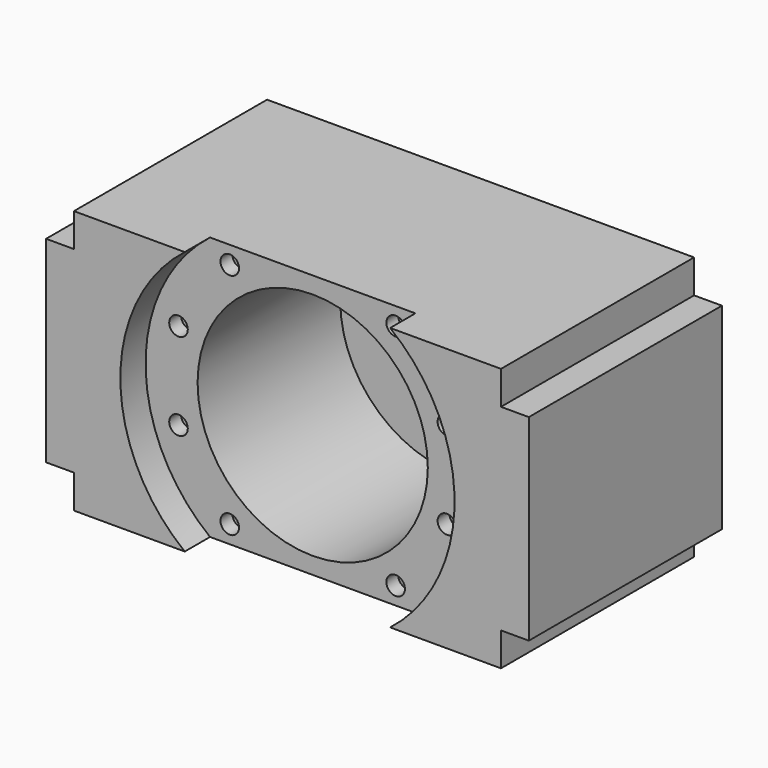
from build123d import *

# Parameters (mm, degrees)
F0_R     = 124
F1_DEPTH = 260
F2_R     = 124
F3_DEPTH = 34
F4_R     = 124
F5_DEPTH = 34
F6_R     = 10
F7_DEPTH = 16


with BuildPart() as f1:
    # F0 (on Front) → F1 (new body)
    with BuildSketch(Plane.XZ):
        Polygon((490, 0), (30, 0), (30, -36), (0, -36), (0, -248), (30, -248), (30, -284), (490, -284), (490, -248), (520, -248), (520, -36), (490, -36), align=None)
        with Locations((260, -142)):
            Circle(F0_R, mode=Mode.SUBTRACT)
    extrude(amount=F1_DEPTH)

    # F2 (on face) → F3 (cut)
    with BuildSketch(Plane.XZ.offset(260)):
        with BuildLine():
            Line((149.3835455278, -284), (370.6164544722, -284))
            ThreePointArc((370.6164544722, -284), (440, -142), (370.6164544722, 0))
            Line((370.6164544722, 0), (149.3835455278, 0))
            ThreePointArc((149.3835455278, 0), (80, -142), (149.3835455278, -284))
        make_face()
        with Locations((260, -142)):
            Circle(F2_R, mode=Mode.SUBTRACT)
    extrude(amount=-F3_DEPTH, mode=Mode.SUBTRACT)

    # F4 (on face) → F5 (join)
    with BuildSketch(Plane(origin=(0, 0, 0), x_dir=(-1, 0, 0), z_dir=(0, 1, 0))):
        Polygon((-30, -36), (-30, 0), (-490, 0), (-490, -36), (-520, -36), (-520, -248), (-490, -248), (-490, -284), (-30, -284), (-30, -248), (0, -248), (0, -36), align=None)
        with Locations((-260, -142)):
            Circle(F4_R, mode=Mode.SUBTRACT)
        with Locations((-260, -142)):
            Circle(F4_R)
    extrude(amount=-F5_DEPTH)

    # F6 (on face) → F7 (cut)
    with BuildSketch(Plane.XZ.offset(226)):
        with Locations((170.6566416515, -19.029416855)):
            Circle(F6_R)
        with Locations((115.4394095231, -95.029416855)):
            Circle(F6_R)
        with Locations((115.4394095231, -188.970583145)):
            Circle(F6_R)
        with Locations((170.6566416515, -264.970583145)):
            Circle(F6_R)
        with Locations((349.3433583485, -264.970583145)):
            Circle(F6_R)
        with Locations((404.5605904769, -188.970583145)):
            Circle(F6_R)
        with Locations((404.5605904769, -95.029416855)):
            Circle(F6_R)
        with Locations((349.3433583485, -19.029416855)):
            Circle(F6_R)
    extrude(amount=-F7_DEPTH, mode=Mode.SUBTRACT)


solid = f1.part
